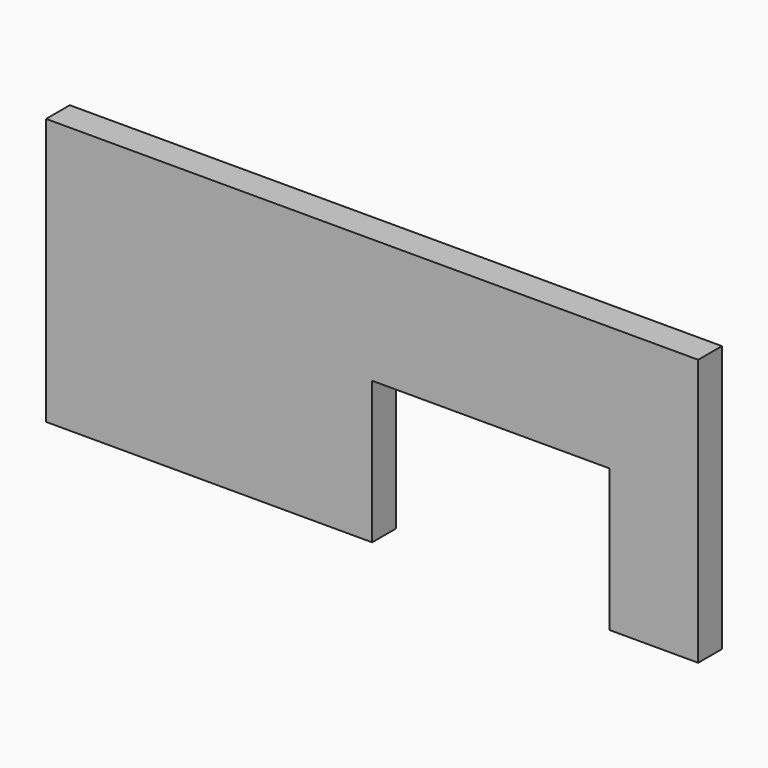
from build123d import *

# Parameters (mm, degrees)
F1_DEPTH = 3.175


# Not quite as in the source:
# - a feature names something its author has since deleted; it is built from what else it names


with BuildPart() as f1:
    # F0 (on Front) → F1 (new body)
    with BuildSketch(Plane.XZ):
        Polygon((12.7, 0), (12.7, -7.62), (22.225, -7.62), (22.225, 20.955), (-47.625, 20.955), (-47.625, -7.62), (-12.7, -7.62), (-12.7, 7.62), (12.7, 7.62), align=None)
    extrude(amount=F1_DEPTH)


solid = f1.part
